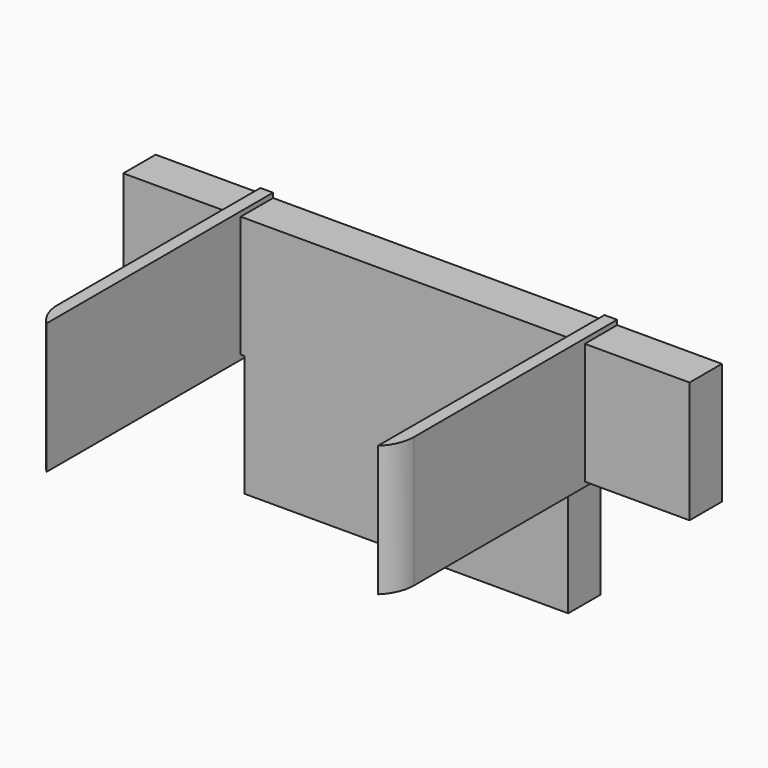
from build123d import *

# Parameters (mm, degrees)
F0_W        = 12.9503121972
F0_H        = 15
F0_R        = 1
F0_W_2      = 1.5692040324
F1_DEPTH    = 5
F2_DEPTH    = 2
F0_H_2      = 0.5759084597
F0_H_3      = 0.5869377777
F3_DEPTH    = 35
F4_T1_DEPTH = 34.3491316119


# Not quite as in the source:
# - a fillet or chamfer that OpenCascade refuses, or shapes differently, is made with other operations: its cross-section is extruded or revolved along the edge and cut away or added
# - a feature names something its author has since deleted; it is built from what else it names


with BuildPart() as f1:
    # F0 (on Front) → F1 (new body)
    with BuildSketch(Plane.XZ):
        with Locations((-28.5248439014, 7.5)):
            Rectangle(F0_W, F0_H)
        Polygon((20.4804837704, 0), (20.4804837704, 15), (-20.4804837704, 15), (-20.4804837704, 0), (-20, 0), (-20, -15), (20, -15), (20, 0), align=None)
        Circle(F0_R, mode=Mode.SUBTRACT)
        with Locations((-21.2650857866, 7.5)):
            Rectangle(F0_W_2, F0_H)
        with Locations((21.2650857866, 7.5)):
            Rectangle(F0_W_2, F0_H)
        with Locations((28.5248439014, 7.5)):
            Rectangle(F0_W, F0_H)
        Circle(F0_R)
    extrude(amount=F1_DEPTH)

    # F0 (on Front) → F2 (join)
    with BuildSketch(Plane.XZ):
        Circle(F0_R)
    extrude(amount=-F2_DEPTH)

    # F0 (on Front) → F3 (join)
    with BuildSketch(Plane.XZ):
        with Locations((-21.2650857866, 7.5)):
            Rectangle(F0_W_2, F0_H)
        with Locations((-21.2650857866, -0.2879542299)):
            Rectangle(F0_W_2, F0_H_2)
        with Locations((-21.2650857866, 15.2934688888)):
            Rectangle(F0_W_2, F0_H_3)
        with Locations((21.2650857866, 15.2934688888)):
            Rectangle(F0_W_2, F0_H_3)
        with Locations((21.2650857866, 7.5)):
            Rectangle(F0_W_2, F0_H)
        with Locations((21.2650857866, -0.2879542299)):
            Rectangle(F0_W_2, F0_H_2)
    extrude(amount=F3_DEPTH)

    # F4: fillet of radius 5 on 2 edges, made by hand

    # F4_s2 → F4_t1 (cut)
    with BuildSketch(Plane.XY.offset(-9.669051147)):
        with BuildLine():
            ThreePointArc((-22.0496878028, -31.3627429251), (-21.6406561014, -33.3434019268), (-20.4804837704, -35))
            Line((-20.4804837704, -35), (-22.0496878028, -35))
            Line((-22.0496878028, -35), (-22.0496878028, -31.3627429251))
        make_face()
        with BuildLine():
            ThreePointArc((20.4804837704, -35), (21.6406561014, -33.3434019268), (22.0496878028, -31.3627429251))
            Line((22.0496878028, -31.3627429251), (22.0496878028, -35))
            Line((22.0496878028, -35), (20.4804837704, -35))
        make_face()
    extrude(amount=F4_T1_DEPTH, mode=Mode.SUBTRACT)


solid = f1.part
